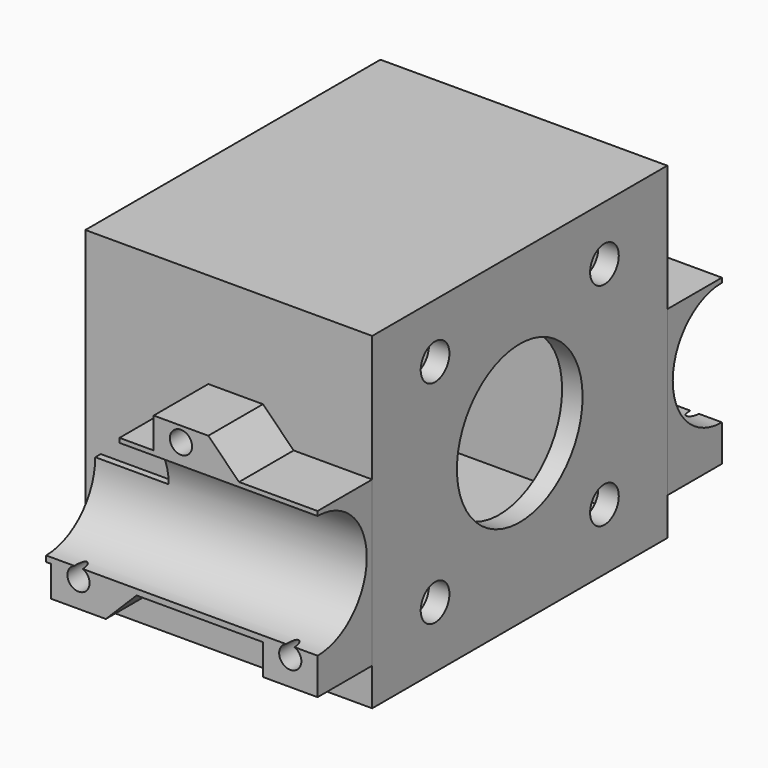
from build123d import *

# Parameters (mm, degrees)
F0_R      = 1.625
F1_DEPTH  = 10
F3_DEPTH  = 39.751
F4_W      = 42
F4_H      = 54
F5_DEPTH  = 48
F6_T      = -3
F9_R      = 2.625
F9_R_2    = 11.5
F10_DEPTH = 42.001


with BuildPart() as f1:
    # F0 (on Front) → F1 (new body)
    with BuildSketch(Plane.XZ):
        Polygon((-5, 5.5), (3, 5.5), (3, 10), (3, 19.85), (3, 29.5), (-8.5, 29.5), (-13, 34), (-21, 34), (-21, 29.5), (-26, 29.5), (-26, 19.85), (-36.75, 19.85), (-36.75, 10), (-36, 10), (-36, 5.5), (-28, 5.5), (-23.5, 10), (-5, 10), align=None)
        with Locations((-32, 9.3499994636)):
            Circle(F0_R, mode=Mode.SUBTRACT)
        with Locations((-1, 9.3499994636)):
            Circle(F0_R, mode=Mode.SUBTRACT)
        with Locations((-17, 31.8499994636)):
            Circle(F0_R, mode=Mode.SUBTRACT)
    extrude(amount=F1_DEPTH)

    # F2 (on face) → F3 (cut, through all)
    with BuildSketch(Plane.YZ.offset(3)):
        with BuildLine():
            Line((-10.3440208091, 28.8434225789), (-10.3440208091, 10.8565774211))
            ThreePointArc((-10.3440208091, 10.8565774211), (-10.1720418405, 10.8516445055), (-10, 10.85))
            Line((-10, 10.85), (-10, 28.85))
            ThreePointArc((-10, 28.85), (-10.1720418405, 28.8483554945), (-10.3440208091, 28.8434225789))
        make_face()
        with BuildLine():
            Line((-10, 28.85), (-10, 10.85))
            ThreePointArc((-10, 10.85), (-1, 19.85), (-10, 28.85))
        make_face()
    extrude(amount=-F3_DEPTH, mode=Mode.SUBTRACT)


with BuildPart() as f5:
    # F4 (on Top) → F5 (new body)
    with BuildSketch(Plane.XY):
        with Locations((-18, 27)):
            Rectangle(F4_W, F4_H)
    extrude(amount=F5_DEPTH)

    # F6
    f6_openings = [f5.faces().sort_by_distance(p)[0] for p in [
        (-39, 27, 24),
    ]]
    offset(amount=F6_T, openings=f6_openings)

    # F9 (on face) → F10 (cut, through all)
    with BuildSketch(Plane.YZ.offset(3)):
        with Locations((11.5, 40)):
            Circle(F9_R)
        with Locations((27, 24.5)):
            Circle(F9_R_2)
        with Locations((11.5, 9)):
            Circle(F9_R)
        with Locations((42.5, 9)):
            Circle(F9_R)
        with Locations((42.5, 40)):
            Circle(F9_R)
    extrude(amount=-F10_DEPTH, mode=Mode.SUBTRACT)


with BuildPart() as f8_1:
    # F8: instance of F1
    add(f1.part.mirror(Plane.XZ.offset(-27)))


solid = Compound([f1.part, f5.part, f8_1.part])
